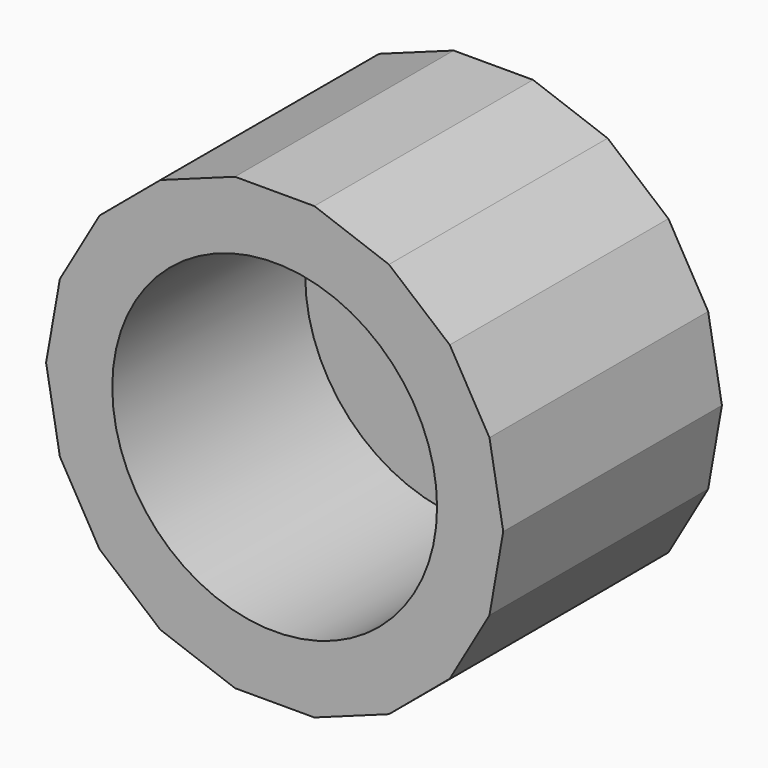
from build123d import *

# Parameters (mm, degrees)
F0_R         = 10.05
F1_DEPTH     = 2
F2_R         = 10.1
F3_DEPTH     = 15
F4_TEXT_SIZE = 4.9312379214
F5_DEPTH     = 1


# Not quite as in the source:
# - Text() gives the source's letters only with a copy of the font that has no kerning and outlines rounded to 1/6400 em; it was checked with that copy


with BuildPart() as f1:
    # F0 (on Front) → F1 (new body)
    with BuildSketch(Plane.XZ):
        Polygon((2.4685777299, 14), (-2.4685777299, 14), (-7.1079862832, 12.311393382), (-10.890066788, 9.1378510253), (-13.3586445179, 4.8621489747), (-14.2159725664, 0), (-13.3586445179, -4.8621489747), (-10.890066788, -9.1378510253), (-7.1079862832, -12.311393382), (-2.4685777299, -14), (2.4685777299, -14), (7.1079862832, -12.311393382), (10.890066788, -9.1378510253), (13.3586445179, -4.8621489747), (14.2159725664, 0), (13.3586445179, 4.8621489747), (10.890066788, 9.1378510253), (7.1079862832, 12.311393382), align=None)
        Circle(F0_R, mode=Mode.SUBTRACT)
        Circle(F0_R)
    extrude(amount=F1_DEPTH)

    # F2 (on face) → F3 (join)
    with BuildSketch(Plane.XZ.offset(2)):
        Polygon((2.4685777299, 14), (-2.4685777299, 14), (-7.1079862832, 12.311393382), (-10.890066788, 9.1378510253), (-13.3586445179, 4.8621489747), (-14.2159725664, 0), (-13.3586445179, -4.8621489747), (-10.890066788, -9.1378510253), (-7.1079862832, -12.311393382), (-2.4685777299, -14), (2.4685777299, -14), (7.1079862832, -12.311393382), (10.890066788, -9.1378510253), (13.3586445179, -4.8621489747), (14.2159725664, 0), (13.3586445179, 4.8621489747), (10.890066788, 9.1378510253), (7.1079862832, 12.311393382), align=None)
        Circle(F2_R, mode=Mode.SUBTRACT)
    extrude(amount=F3_DEPTH)

    # F4 (on face) → F5 (join)
    with BuildSketch(Plane(origin=(-4.7882820066, 0, -13.155696691), x_dir=(0.9396926208, 0, -0.3420201433), z_dir=(-0.3420201433, 0, -0.9396926208))):
        with Locations((-1.1280206745, 12.2500355355)):
            Text('*', F4_TEXT_SIZE, font='Arimo', font_style=FontStyle.BOLD, text_align=(TextAlign.LEFT, TextAlign.BOTTOM))
        with Locations((-1.1280206745, 6.579111926)):
            Text('*', F4_TEXT_SIZE, font='Arimo', font_style=FontStyle.BOLD, text_align=(TextAlign.LEFT, TextAlign.BOTTOM))
        with Locations((-1.1280206745, 0.9081883164)):
            Text('*', F4_TEXT_SIZE, font='Arimo', font_style=FontStyle.BOLD, text_align=(TextAlign.LEFT, TextAlign.BOTTOM))
    extrude(amount=F5_DEPTH)


solid = f1.part
